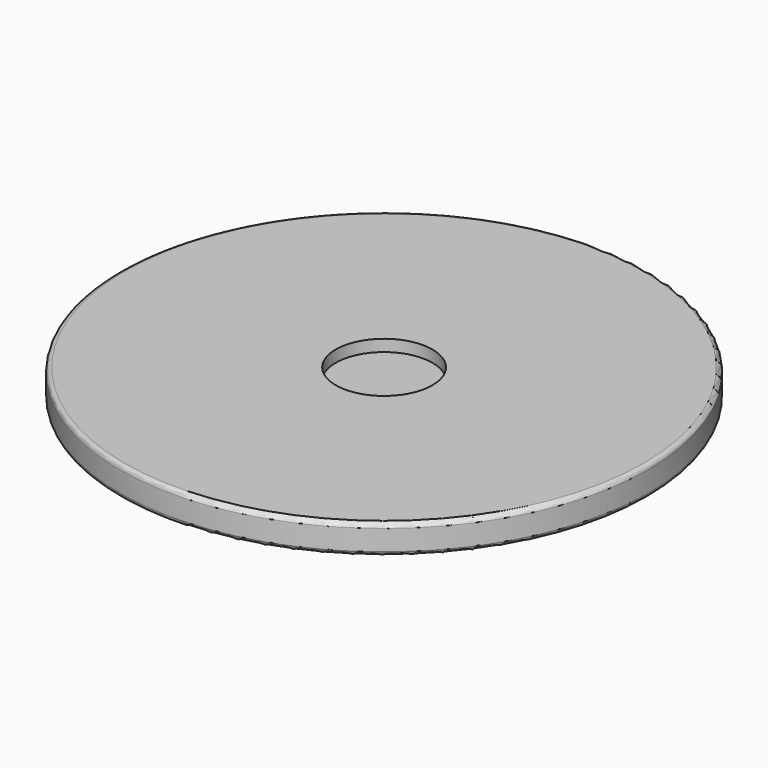
from build123d import *

# Parameters (mm, degrees)
F0_R     = 9
F1_DEPTH = 1
F2_R     = 0.15
F3_R     = 1.65
F4_DEPTH = 0.4


# Not quite as in the source:
# - a feature names something its author has since deleted; it is built from what else it names


with BuildPart() as f1:
    # F0 (on Top) → F1 (new body)
    with BuildSketch(Plane.XY):
        Circle(F0_R)
    extrude(amount=F1_DEPTH)

    # F2
    f2_edges = [f1.edges().sort_by_distance(p)[0] for p in [
        (-9, 0, 1),
        (-9, 0, 0),
    ]]
    fillet(f2_edges, radius=F2_R)

    # F3 (on face) → F4 (cut)
    with BuildSketch(Plane.XY.offset(1)):
        Circle(F3_R)
    extrude(amount=-F4_DEPTH, mode=Mode.SUBTRACT)


solid = f1.part
